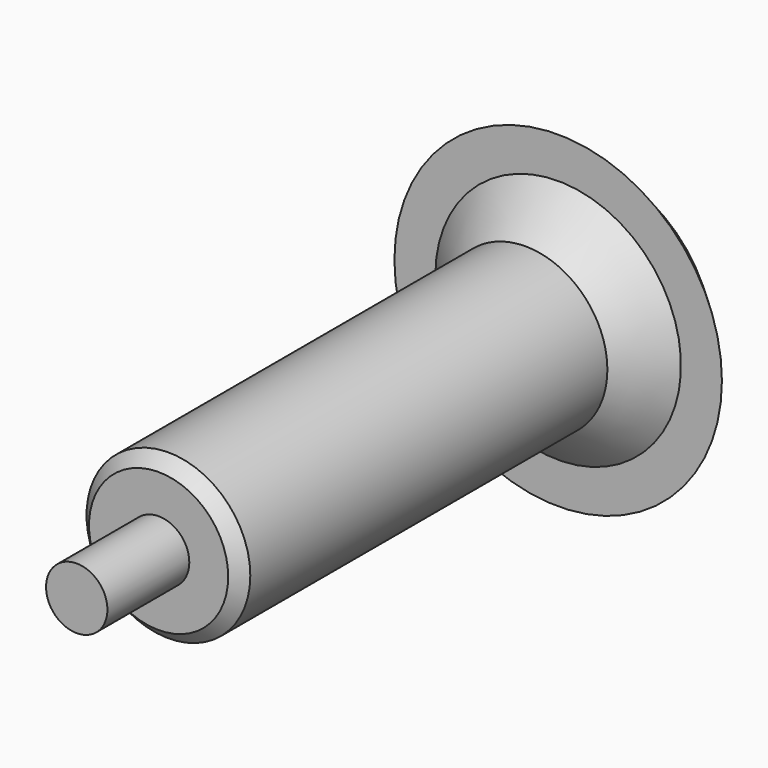
from build123d import *

# Parameters (mm, degrees)
F0_R     = 20
F1_DEPTH = 112
F2_SIZE  = 3
F3_R     = 7.5
F4_DEPTH = 25
F5_R     = 30
F6_DEPTH = 10
F7_SIZE  = 9.99999
F8_R     = 40
F9_DEPTH = 10
F10_SIZE = 9.99999


# Not quite as in the source:
# - a fillet or chamfer is up to 0.001 mm smaller than in the source, because OpenCascade refuses the exact size


with BuildPart() as f1:
    # F0 (on Front) → F1 (new body)
    with BuildSketch(Plane.XZ):
        Circle(F0_R)
    extrude(amount=F1_DEPTH)

    # F2
    f2_edges = [f1.edges().sort_by_distance(p)[0] for p in [
        (-20, -112, 0),
    ]]
    chamfer(f2_edges, length=F2_SIZE)

    # F3 (on face) → F4 (join)
    with BuildSketch(Plane.XZ.offset(112)):
        Circle(F3_R)
    extrude(amount=F4_DEPTH)

    # F5 (on face) → F6 (join)
    with BuildSketch(Plane(origin=(0, 0, 0), x_dir=(-1, 0, 0), z_dir=(0, 1, 0))):
        Circle(F5_R)
    extrude(amount=F6_DEPTH)

    # F7 (size 10 in the source; OpenCascade refuses exactly that, so slightly less here)
    f7_edges = [f1.edges().sort_by_distance(p)[0] for p in [
        (30, 0, 0),
    ]]
    chamfer(f7_edges, length=F7_SIZE)

    # F8 (on face) → F9 (join)
    with BuildSketch(Plane(origin=(0, 10, 0), x_dir=(-1, 0, 0), z_dir=(0, 1, 0))):
        Circle(F8_R)
    extrude(amount=F9_DEPTH)

    # F10 (size 10 in the source; OpenCascade refuses exactly that, so slightly less here)
    f10_edges = [f1.edges().sort_by_distance(p)[0] for p in [
        (40, 20, 0),
    ]]
    chamfer(f10_edges, length=F10_SIZE)


solid = f1.part
